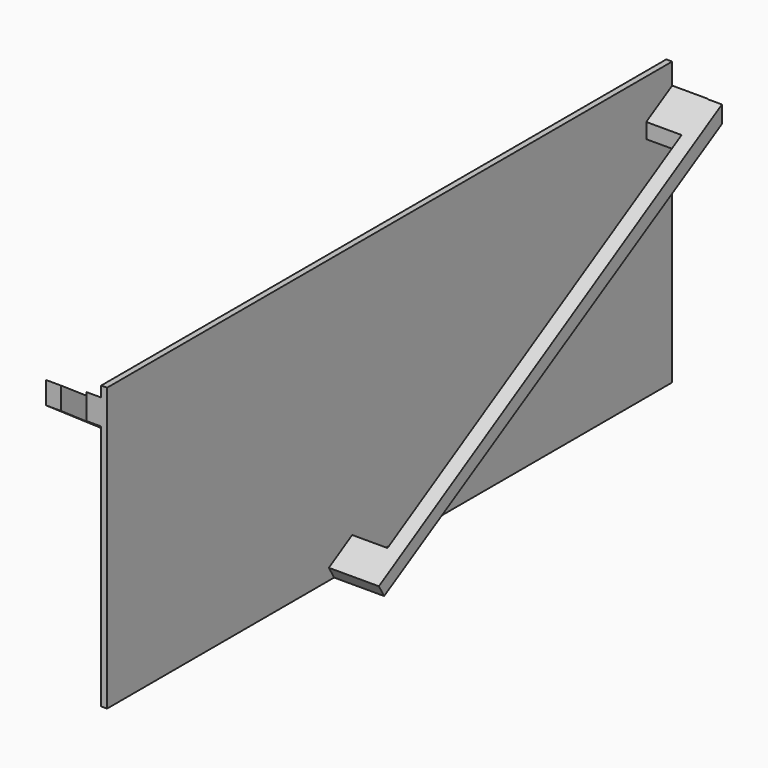
from build123d import *

# Parameters (mm, degrees)
F0_W      = 6096
F0_H      = 2438.4
F1_DEPTH  = 50.8
F3_DEPTH  = 304.8
F5_DEPTH  = 127
F7_DEPTH  = 203.2
F10_DEPTH = 127
F12_DEPTH = 127


with BuildPart() as f1:
    # F0 (on Right) → F1 (new body)
    with BuildSketch(Plane.YZ):
        Rectangle(F0_W, F0_H)
    extrude(amount=F1_DEPTH)

    # F2 (on face) → F3 (join)
    with BuildSketch(Plane.YZ.offset(50.8)):
        Polygon((2768.7226924944, 742.9208226702), (3048, 905.6503176689), (3048, 1036.5047400729), (2768.7226924944, 873.7752450741), align=None)
        Polygon((-655.6012799492, -1121.512219292), (-598.6804962158, -1219.2), (-403.7681643359, -1105.6283474403), (-403.7681643359, -974.7739250363), align=None)
    extrude(amount=F3_DEPTH)

    # F4 (on face) → F5 (join)
    with BuildSketch(Plane(origin=(0, 0, 0), x_dir=(0, -1, 0), z_dir=(-1, 0, 0))):
        Polygon((0, -1219.2), (3048, 908.1615209579), (3048, 1128.1091420174), (0, -999.2523789406), align=None)
    extrude(amount=F5_DEPTH)

    # F6 (on face) → F7 (join)
    with BuildSketch(Plane(origin=(-127, 0, 0), x_dir=(0, -1, 0), z_dir=(-1, 0, 0))):
        Polygon((611.3445986138, -572.562426468), (184.8353640356, -870.2459349899), (184.8353640356, -1090.1935560493), (611.3445986138, -792.5100475274), align=None)
    extrude(amount=F7_DEPTH)

    # F9 (on face) → F10 (join)
    with BuildSketch(Plane(origin=(-330.2, 0, 0), x_dir=(0, -1, 0), z_dir=(-1, 0, 0))):
        Polygon((0, -986.7016077042), (0, -1209.7096443176), (184.8353640356, -1080.9821333739), (184.8353640356, -870.2459349899), (611.3445986138, -572.562426468), (611.3445986138, -783.9422652285), (3071.0999965668, 929.1400313377), (3071.0999965668, 1121.7379570007), align=None)
        Polygon((184.8353640356, -870.2459349899), (184.8353640356, -1080.9821333739), (611.3445986138, -783.9422652285), (611.3445986138, -572.562426468), align=None)
    extrude(amount=F10_DEPTH)

    # F11 (on face) → F12 (join)
    with BuildSketch(Plane.YZ.offset(355.6)):
        Polygon((3045.1943140363, 1034.869921032), (-655.6012799492, -1121.512219292), (-598.6804962158, -1219.2), (3045.1943140363, 886.5033388138), align=None)
    extrude(amount=F12_DEPTH)


solid = f1.part
